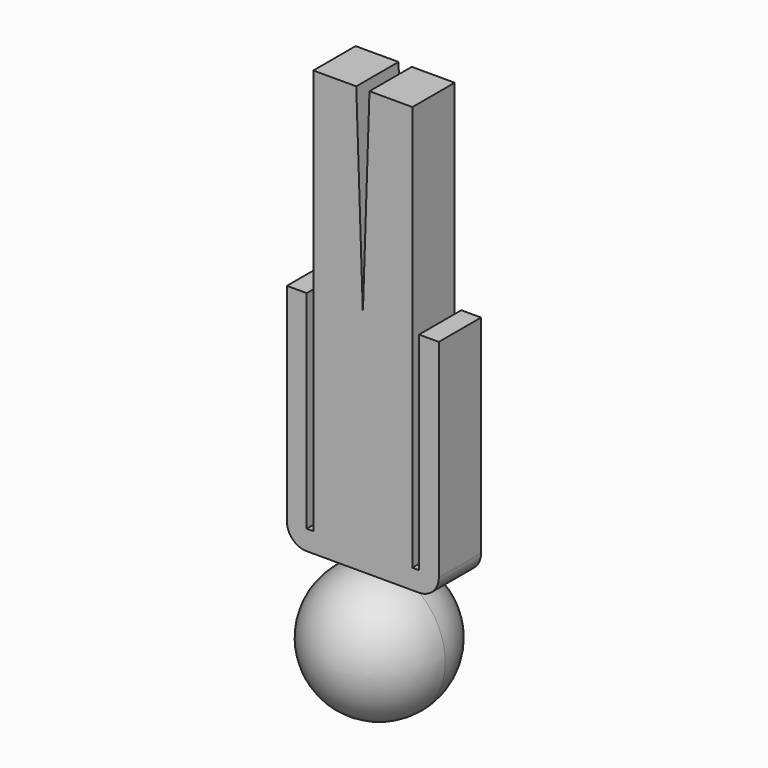
from build123d import *

# Parameters (mm, degrees)
F0_R          = 25.4
F1_DEPTH      = 50.8
F2_R          = 25.4
F3_R          = 25.39999
F4_W          = 7.62
F4_H          = 10.16
F4_W_2        = 7.6200046011
F5_DEPTH      = 50.8
F6_W          = 21.59
F6_H          = 14.5421422695
F7_DEPTH      = 61.976
F7_DEPTH_BACK = 25.4
F8_R          = 7.62
F9_R          = 7.62
F10_W         = 2.54
F10_H         = 79.756
F11_DEPTH     = 25.4
F12_W         = 38.1
F12_H         = 20.32
F13_DEPTH     = 76.2
F15_DEPTH     = 25.4


# Not quite as in the source:
# - a fillet or chamfer is up to 0.001 mm smaller than in the source, because OpenCascade refuses the exact size


with BuildPart() as f1:
    # F0 (on Front) → F1 (new body)
    with BuildSketch(Plane.XZ):
        Circle(F0_R)
    extrude(amount=F1_DEPTH)

    # F2
    f2_edges = [f1.edges().sort_by_distance(p)[0] for p in [
        (-25.4, -50.8, 0),
    ]]
    fillet(f2_edges, radius=F2_R)

    # F3 (radius 25.4 in the source; OpenCascade refuses exactly that, so slightly less here)
    f3_edges = [f1.edges().sort_by_distance(p)[0] for p in [
        (-25.4, 0, 0),
    ]]
    fillet(f3_edges, radius=F3_R)

    # F4 (on Top) → F5 (join)
    with BuildSketch(Plane.XY):
        with Locations((3.81, -23.7836401282)):
            Rectangle(F4_W, F4_H)
        with Locations((-3.8100023006, -23.7836401282)):
            Rectangle(F4_W_2, F4_H)
    extrude(amount=F5_DEPTH)

    # F6 (on face) → F7 (join, two sides)
    with BuildSketch(Plane.XY.offset(50.8)) as f7_sk:
        Polygon((7.62, -33.2457823977), (7.62, -18.7036401282), (29.21, -18.7036401282), (29.21, -12.9257823977), (-29.21, -12.9257823977), (-29.21, -18.7036401282), (-29.21, -33.2457823977), align=None)
        with Locations((18.415, -25.9747112629)):
            Rectangle(F6_W, F6_H)
    extrude(amount=F7_DEPTH)
    extrude(f7_sk.sketch, amount=-F7_DEPTH_BACK)

    # F8
    f8_edges = [f1.edges().sort_by_distance(p)[0] for p in [
        (29.21, -23.085782, 25.4),
    ]]
    fillet(f8_edges, radius=F8_R)

    # F9
    f9_edges = [f1.edges().sort_by_distance(p)[0] for p in [
        (-29.21, -23.085782, 25.4),
    ]]
    fillet(f9_edges, radius=F9_R)

    # F10 (on face) → F11 (cut)
    with BuildSketch(Plane.XZ.offset(33.2457823977)):
        with Locations((20.32, 72.898)):
            Rectangle(F10_W, F10_H)
        with Locations((-20.32, 72.898)):
            Rectangle(F10_W, F10_H)
    extrude(amount=-F11_DEPTH, mode=Mode.SUBTRACT)

    # F12 (on face) → F13 (join)
    with BuildSketch(Plane.XY.offset(112.776)):
        with Locations((0, -23.0857823977)):
            Rectangle(F12_W, F12_H)
    extrude(amount=F13_DEPTH)

    # F14 (on face) → F15 (cut)
    with BuildSketch(Plane(origin=(0, -12.9257823977, 0), x_dir=(-1, 0, 0), z_dir=(0, 1, 0))):
        Polygon((-2.54, 188.976), (0, 112.776), (0, 188.976), align=None)
        Polygon((0, 188.976), (0, 112.776), (2.54, 188.976), align=None)
    extrude(amount=-F15_DEPTH, mode=Mode.SUBTRACT)


solid = f1.part
